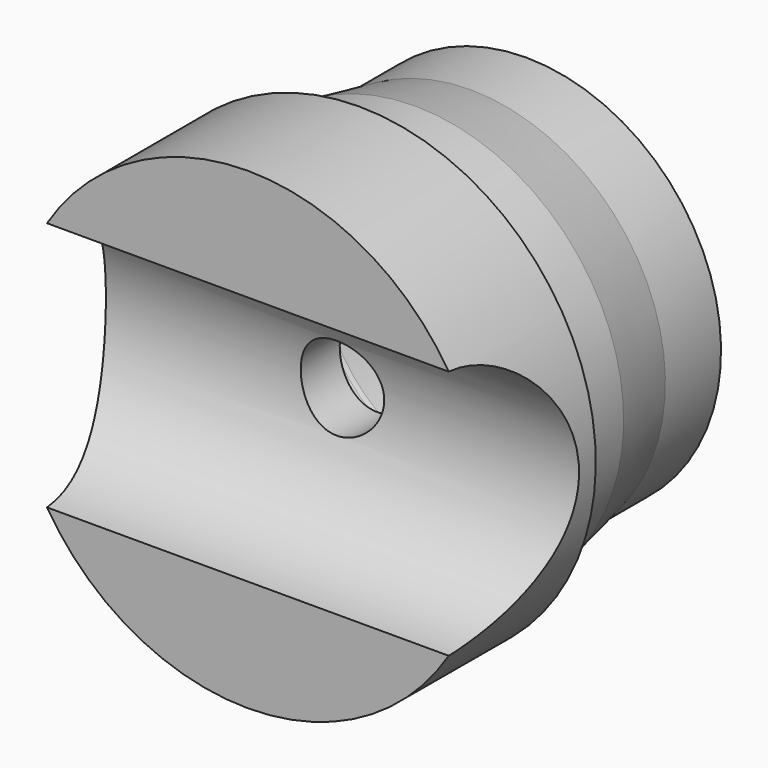
from build123d import *

# Parameters (mm, degrees)
F2_R     = 9
F3_DEPTH = 25
F5_T     = 3.5
F6_D     = 6


# Not quite as in the source:
# - a shell that OpenCascade refuses in one call is made with other operations: the cavity is built on its own and cut out


with BuildPart() as f1:
    # F0 (on Right) → F1 (revolve)
    with BuildSketch(Plane.YZ):
        Polygon((0, 0), (25, 0), (25, 14), (20, 14), (15, 15), (10, 15), (10, 17), (0, 17), align=None)
    revolve(axis=Axis((0, 12.5, 0), (0, 1, 0)))

    # F2 (on Right) → F3 (cut, symmetric)
    with BuildSketch(Plane.YZ):
        with Locations((-0.5, 0)):
            Circle(F2_R)
    extrude(amount=F3_DEPTH, both=True, mode=Mode.SUBTRACT)

    # F5: shell of thickness 3.5, made by hand


with BuildPart() as f5_core1:
    # F5_t2: copy of F1
    add(f1.part)

    # the walls: a layer under each face that stays
    f5_faces = [f5_core1.faces().sort_by_distance(p)[0] for p in [
        (0, 22.5, -14),
        (0, 17.5, -14.5),
        (0, 12.5, -15),
        (-11.3333333333, 10, 11.3333333333),
        (0, 5, -17),
        (0, 0, -12.9930501889),
        (0, 8.5, 0),
        (0, 0, 12.9930501889),
    ]]
    thicken(f5_faces, amount=-F5_T, mode=Mode.SUBTRACT)

    # F5_s3 → F5_t4 (revolve, cut)
    with BuildSketch(Plane.YZ):
        Polygon((20.0068640647, 14.0693203236), (20, 10.5), (19.6534317024, 10.5), (19.313593527, 10.5679676351), align=None)
    revolve(axis=Axis((0, 20, 0), (0, 1, 0)), mode=Mode.SUBTRACT)

    # F5_s5 → F5_t6 (revolve, cut)
    with BuildSketch(Plane.YZ):
        Polygon((10.035, 15.035), (10, 11.5), (6.5, 11.5), (6.5, 15), align=None)
    revolve(axis=Axis((0, 10, 0), (0, 1, 0)), mode=Mode.SUBTRACT)


with BuildPart() as f1_1:
    add(f1.part)

    # what is left inside the walls is the cavity
    f5_cavity = [f5_core1.part.solids().sort_by_distance(p)[0] for p in [
        (-3.834029, 12.035, 0),
    ]]
    add(f5_cavity, mode=Mode.SUBTRACT)

    # F6 (through all)
    with Locations(Plane(origin=(0, 25, 0), x_dir=(-1, 0, 0), z_dir=(0, 1, 0))):
        with Locations((0, 0)):
            Hole(F6_D / 2)


solid = f1_1.part
